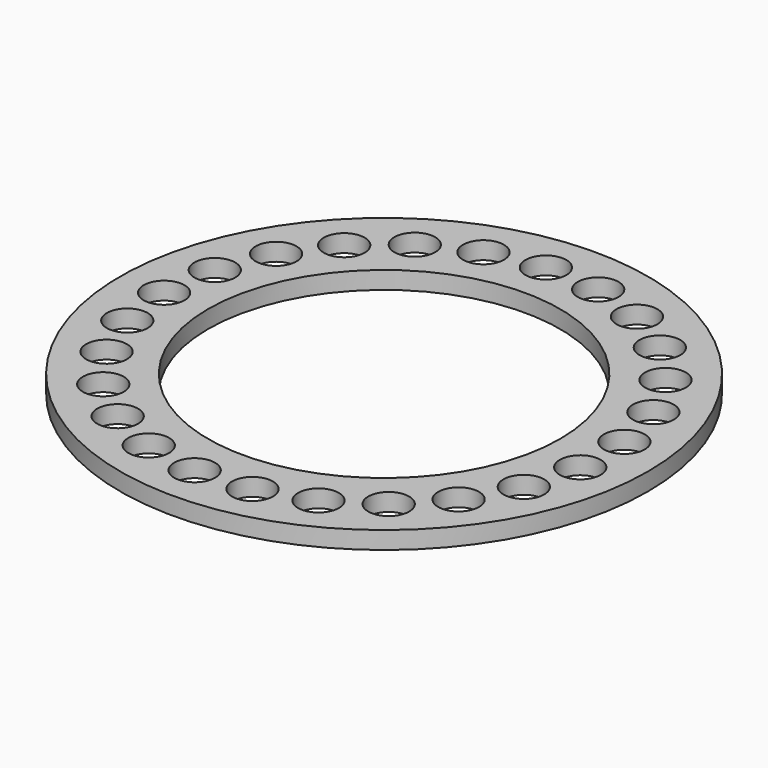
from build123d import *

# Parameters (mm, degrees)
F0_R     = 3810
F0_R_2   = 294.9557001393
F0_R_3   = 2540
F1_DEPTH = 127


# Not quite as in the source:
# - a feature names something its author has since deleted; it is built from what else it names


with BuildPart() as f1:
    # F0 (on Top) → F1 (new body, symmetric)
    with BuildSketch(Plane.XY):
        Circle(F0_R)
        with Locations((-2314.475392063, -2173.4370613236)):
            Circle(F0_R_2, mode=Mode.SUBTRACT)
        with Locations((-981.1289571405, -3019.6044392371)):
            Circle(F0_R_2, mode=Mode.SUBTRACT)
        with Locations((-199.3598995056, -3168.7348627598)):
            Circle(F0_R_2, mode=Mode.SUBTRACT)
        with Locations((-1701.2500740583, -2680.7411634689)):
            Circle(F0_R_2, mode=Mode.SUBTRACT)
        with Locations((-2782.2737091393, -1529.5679152729)):
            Circle(F0_R_2, mode=Mode.SUBTRACT)
        with Locations((-3075.2515365834, -789.5903917484)):
            Circle(F0_R_2, mode=Mode.SUBTRACT)
        with Locations((594.9356738097, -3118.7620210636)):
            Circle(F0_R_2, mode=Mode.SUBTRACT)
        with Locations((1351.8492507191, -2872.8258915796)):
            Circle(F0_R_2, mode=Mode.SUBTRACT)
        with Locations((2023.8211674521, -2446.3795458131)):
            Circle(F0_R_2, mode=Mode.SUBTRACT)
        with Locations((2568.6289571405, -1866.2181760286)):
            Circle(F0_R_2, mode=Mode.SUBTRACT)
        with Locations((2952.0403426952, -1168.7954547739)):
            Circle(F0_R_2, mode=Mode.SUBTRACT)
        with Locations((3149.9641766735, -397.9330165667)):
            Circle(F0_R_2, mode=Mode.SUBTRACT)
        with Locations((-3175, 0)):
            Circle(F0_R_2, mode=Mode.SUBTRACT)
        with Locations((-3075.2515365834, 789.5903917484)):
            Circle(F0_R_2, mode=Mode.SUBTRACT)
        with Locations((-2782.2737091393, 1529.5679152729)):
            Circle(F0_R_2, mode=Mode.SUBTRACT)
        with Locations((-2314.475392063, 2173.4370613236)):
            Circle(F0_R_2, mode=Mode.SUBTRACT)
        with Locations((-1701.2500740583, 2680.7411634689)):
            Circle(F0_R_2, mode=Mode.SUBTRACT)
        with Locations((-981.1289571405, 3019.6044392371)):
            Circle(F0_R_2, mode=Mode.SUBTRACT)
        with Locations((-199.3598995056, 3168.7348627598)):
            Circle(F0_R_2, mode=Mode.SUBTRACT)
        Circle(F0_R_3, mode=Mode.SUBTRACT)
        with Locations((3149.9641766735, 397.9330165667)):
            Circle(F0_R_2, mode=Mode.SUBTRACT)
        with Locations((2568.6289571405, 1866.2181760286)):
            Circle(F0_R_2, mode=Mode.SUBTRACT)
        with Locations((2952.0403426952, 1168.7954547739)):
            Circle(F0_R_2, mode=Mode.SUBTRACT)
        with Locations((594.9356738097, 3118.7620210636)):
            Circle(F0_R_2, mode=Mode.SUBTRACT)
        with Locations((1351.8492507191, 2872.8258915796)):
            Circle(F0_R_2, mode=Mode.SUBTRACT)
        with Locations((2023.8211674521, 2446.3795458131)):
            Circle(F0_R_2, mode=Mode.SUBTRACT)
    extrude(amount=F1_DEPTH, both=True)


solid = f1.part
